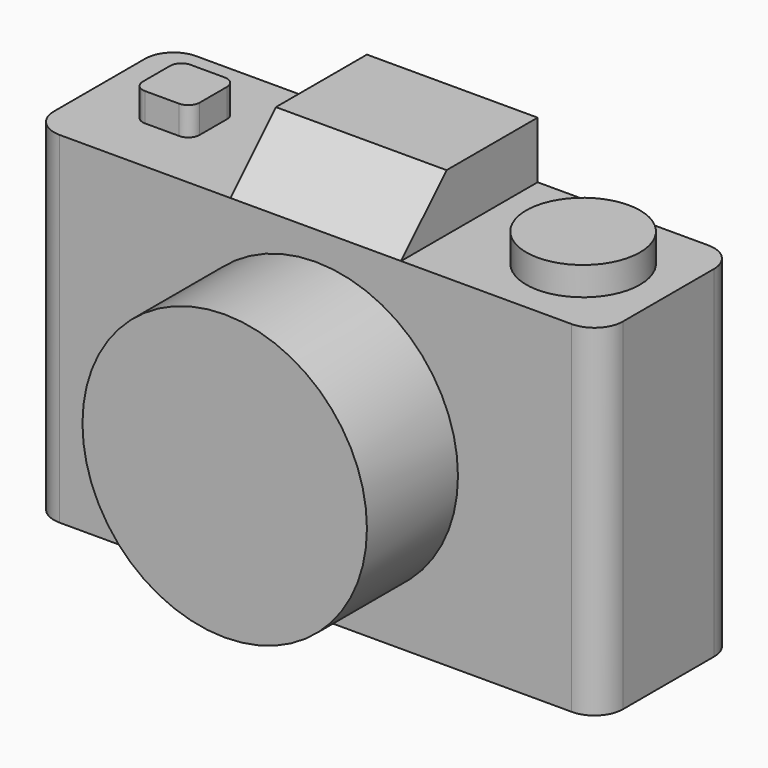
from build123d import *

# Parameters (mm, degrees)
F0_W          = 100
F0_H          = 30
F1_DEPTH      = 60
F2_R          = 10
F2_W          = 10
F2_H          = 10
F3_DEPTH      = 5
F4_R          = 25
F5_DEPTH      = 20
F8_DEPTH      = 30
F9_R          = 5
F10_W         = 79.245492816
F10_H         = 38.8751035929
F11_DEPTH     = 3
F12_R         = 2
F13_TEXT_SIZE = 13.8525980421
F14_DEPTH     = 2


# Not quite as in the source:
# - Text() gives the source's letters only with a copy of the font that has no kerning and outlines rounded to 1/6400 em; it was checked with that copy


with BuildPart() as f1:
    # F0 (on Top) → F1 (new body)
    with BuildSketch(Plane.XY):
        Rectangle(F0_W, F0_H)
    extrude(amount=F1_DEPTH)

    # F2 (on face) → F3 (join)
    with BuildSketch(Plane.XY.offset(60)):
        with Locations((35, 0)):
            Circle(F2_R)
        with Locations((-35, 0)):
            Rectangle(F2_W, F2_H)
    extrude(amount=F3_DEPTH)

    # F4 (on face) → F5 (join)
    with BuildSketch(Plane.XZ.offset(15)):
        with Locations((0, 30)):
            Circle(F4_R)
    extrude(amount=F5_DEPTH)

    # F7 (on offset) → F8 (join)
    with BuildSketch(Plane.YZ.offset(15)):
        Polygon((-5.0000180304, 69.9999092519), (-15.0000180304, 59.9999092519), (14.9999819696, 59.9999092519), (14.9999819696, 69.9999092519), align=None)
    extrude(amount=-F8_DEPTH)

    # F9
    f9_edges = [f1.edges().sort_by_distance(p)[0] for p in [
        (50, -15, 30),
        (50, 15, 30),
        (-50, 15, 30),
        (-50, -15, 30),
    ]]
    fillet(f9_edges, radius=F9_R)

    # F10 (on face) → F11 (cut)
    with BuildSketch(Plane(origin=(0, 15, 0), x_dir=(-1, 0, 0), z_dir=(0, 1, 0))):
        with Locations((0, 34.4375517964)):
            Rectangle(F10_W, F10_H)
    extrude(amount=-F11_DEPTH, mode=Mode.SUBTRACT)

    # F12
    f12_edges = [f1.edges().sort_by_distance(p)[0] for p in [
        (-40, 5, 62.5),
        (-40, -5, 62.5),
        (-30, -5, 62.5),
        (-30, 5, 62.5),
    ]]
    fillet(f12_edges, radius=F12_R)

    # F13 (on face) → F14 (join)
    with BuildSketch(Plane(origin=(0, 15, 0), x_dir=(-1, 0, 0), z_dir=(0, 1, 0))):
        with Locations((-42.6980555058, 2.5538858026)):
            Text('NIKON FIKRI', F13_TEXT_SIZE, font='Open Sans', font_style=FontStyle.BOLD, text_align=(TextAlign.LEFT, TextAlign.BOTTOM))
    extrude(amount=F14_DEPTH)


solid = f1.part
